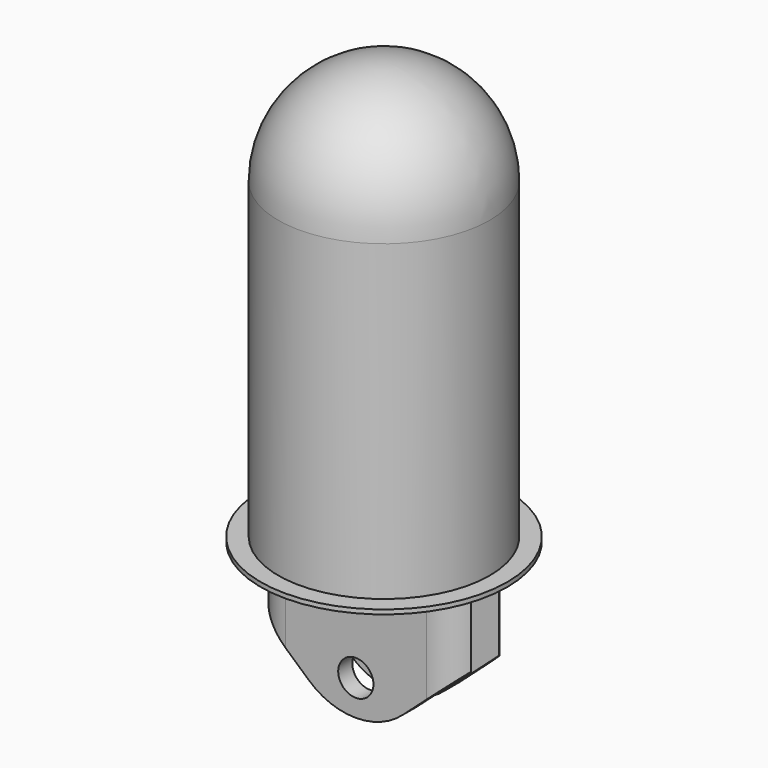
from build123d import *

# Parameters (mm, degrees)
F0_R        = 38.1
F1_DEPTH    = 152.4
F2_R        = 38.1
F4_DEPTH    = 12.7
F5_T1_DEPTH = 57.15
F6_W        = 12.7
F6_H        = 50.8
F7_DEPTH    = 38.1
F0_R_2      = 44.45
F8_DEPTH    = 1.5875


# Not quite as in the source:
# - a fillet or chamfer that OpenCascade refuses, or shapes differently, is made with other operations: its cross-section is extruded or revolved along the edge and cut away or added


with BuildPart() as f1:
    # F0 (on Top) → F1 (new body)
    with BuildSketch(Plane.XY):
        Circle(F0_R)
    extrude(amount=F1_DEPTH)

    # F2
    f2_edges = [f1.edges().sort_by_distance(p)[0] for p in [
        (-38.1, 0, 152.4),
    ]]
    fillet(f2_edges, radius=F2_R)

    # F3 (on Front) → F4 (join, symmetric)
    with BuildSketch(Plane.XZ):
        with BuildLine():
            Line((16.9333333333, -44.3320422095), (38.1, -25.4))
            Line((38.1, -25.4), (38.1, 0))
            Line((38.1, 0), (0, 0))
            Line((0, 0), (-38.1, 0))
            Line((-38.1, 0), (-38.1, -25.4))
            Line((-38.1, -25.4), (-16.9333333333, -44.3320422095))
            ThreePointArc((-16.9333333333, -44.3320422095), (0, -50.8), (16.9333333333, -44.3320422095))
        make_face()
        with BuildLine():
            ThreePointArc((6.35, -38.1), (-4.4901280605, -42.5901280605), (0, -31.75))
            ThreePointArc((0, -31.75), (4.4901280605, -33.6098719395), (6.35, -38.1))
        make_face(mode=Mode.SUBTRACT)
    extrude(amount=F4_DEPTH, both=True)

    # F5: fillet of radius 12.7 on 4 edges, made by hand

    # F5_s2 → F5_t1 (cut)
    with BuildSketch(Plane.XY.offset(-57.15)):
        with BuildLine():
            ThreePointArc((38.1, 0), (34.3802561211, -8.9802561211), (25.4, -12.7))
            Line((25.4, -12.7), (38.1, -12.7))
            Line((38.1, -12.7), (38.1, 0))
        make_face()
        with BuildLine():
            ThreePointArc((38.1, 0), (34.3802561211, 8.9802561211), (25.4, 12.7))
            Line((25.4, 12.7), (38.1, 12.7))
            Line((38.1, 12.7), (38.1, 0))
        make_face()
        with BuildLine():
            ThreePointArc((-25.4, 12.7), (-34.3802561211, 8.9802561211), (-38.1, 0))
            Line((-38.1, 0), (-38.1, 12.7))
            Line((-38.1, 12.7), (-25.4, 12.7))
        make_face()
        with BuildLine():
            ThreePointArc((-38.1, 0), (-34.3802561211, -8.9802561211), (-25.4, -12.7))
            Line((-25.4, -12.7), (-38.1, -12.7))
            Line((-38.1, -12.7), (-38.1, 0))
        make_face()
    extrude(amount=F5_T1_DEPTH, mode=Mode.SUBTRACT)

    # F6 (on Right) → F7 (cut, symmetric)
    with BuildSketch(Plane.YZ):
        with Locations((0, -25.4)):
            Rectangle(F6_W, F6_H)
    extrude(amount=F7_DEPTH, both=True, mode=Mode.SUBTRACT)

    # F0 (on Top) → F8 (join)
    with BuildSketch(Plane.XY):
        Circle(F0_R_2)
        Circle(F0_R, mode=Mode.SUBTRACT)
    extrude(amount=F8_DEPTH)


solid = f1.part
